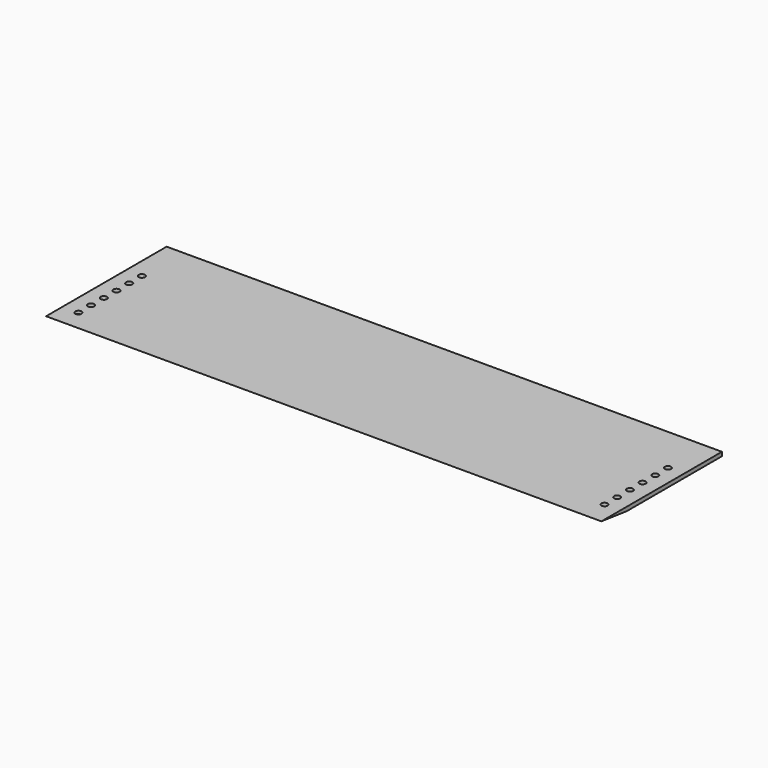
from build123d import *

# Parameters (mm, degrees)
F0_W     = 444.5
F0_H     = 127
F1_DEPTH = 3.175
F2_R     = 2.5527
F2_R_2   = 2.4892
F3_DEPTH = 25.4
F5_DEPTH = 444.501


# Not quite as in the source:
# - a feature names something its author has since deleted; it is built from what else it names


with BuildPart() as f1:
    # F0 (on Top) → F1 (new body)
    with BuildSketch(Plane.XY):
        with Locations((222.25, -63.5)):
            Rectangle(F0_W, F0_H)
    extrude(amount=F1_DEPTH)

    # F2 (on face) → F3 (cut)
    with BuildSketch(Plane.XY.offset(3.175)):
        with Locations((12.7, -104.1527)):
            Circle(F2_R)
        with Locations((12.7, -91.4527)):
            Circle(F2_R)
        with Locations((12.7, -78.7527)):
            Circle(F2_R)
        with Locations((12.7, -66.0527)):
            Circle(F2_R)
        with Locations((12.7, -53.3527)):
            Circle(F2_R)
        with Locations((431.8, -101.6)):
            Circle(F2_R_2)
        with Locations((431.8, -88.9)):
            Circle(F2_R_2)
        with Locations((431.8, -76.2)):
            Circle(F2_R_2)
        with Locations((431.8, -63.5)):
            Circle(F2_R_2)
        with Locations((431.8, -50.8)):
            Circle(F2_R_2)
        with Locations((12.7, -40.6527)):
            Circle(F2_R)
        with Locations((431.8, -38.1)):
            Circle(F2_R_2)
    extrude(amount=-F3_DEPTH, mode=Mode.SUBTRACT)

    # F4 (on face) → F5 (cut, through all)
    with BuildSketch(Plane.YZ.offset(444.5)):
        Polygon((-95.25, 0), (-120.65, 3.175), (-127, 3.175), (-127, 0), align=None)
    extrude(amount=-F5_DEPTH, mode=Mode.SUBTRACT)


solid = f1.part
